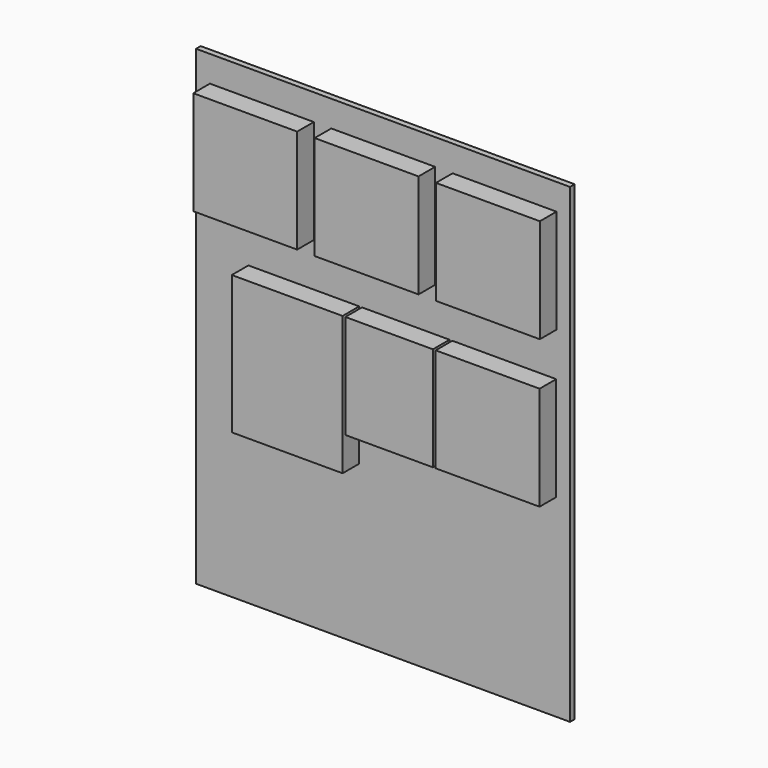
from build123d import *

# Parameters (mm, degrees)
F0_W     = 342.9
F0_H     = 431.8
F1_DEPTH = 5.334
F2_W     = 95.25
F2_H     = 95.25
F2_W_2   = 80.27
F3_DEPTH = 19.05


# Not quite as in the source:
# - a feature names something its author has since deleted; it is built from what else it names


with BuildPart() as f1:
    # F0 (on Front) → F1 (new body)
    with BuildSketch(Plane.XZ):
        with Locations((-26.3048716933, -22.2786769863)):
            Rectangle(F0_W, F0_H)
    extrude(amount=F1_DEPTH)

    # F2 (on face) → F3 (join)
    with BuildSketch(Plane.XZ.offset(5.334)):
        with Locations((-137.4298716933, 121.9963230137)):
            Rectangle(F2_W, F2_H)
        with Locations((-26.1798716933, 121.9963230137)):
            Rectangle(F2_W, F2_H)
        with Locations((85.0701283067, 121.9963230137)):
            Rectangle(F2_W, F2_H)
        Polygon((-48.1548716933, 34.3713230137), (-149.7548716933, 34.3713230137), (-149.7548716933, -92.6286769863), (-48.1548716933, -92.6286769863), (-48.1548716933, -60.8786769863), align=None)
        with Locations((-5.4798716933, -13.2536769863)):
            Rectangle(F2_W_2, F2_H)
        with Locations((84.8201283067, -13.2536769863)):
            Rectangle(F2_W, F2_H)
    extrude(amount=F3_DEPTH)


solid = f1.part
